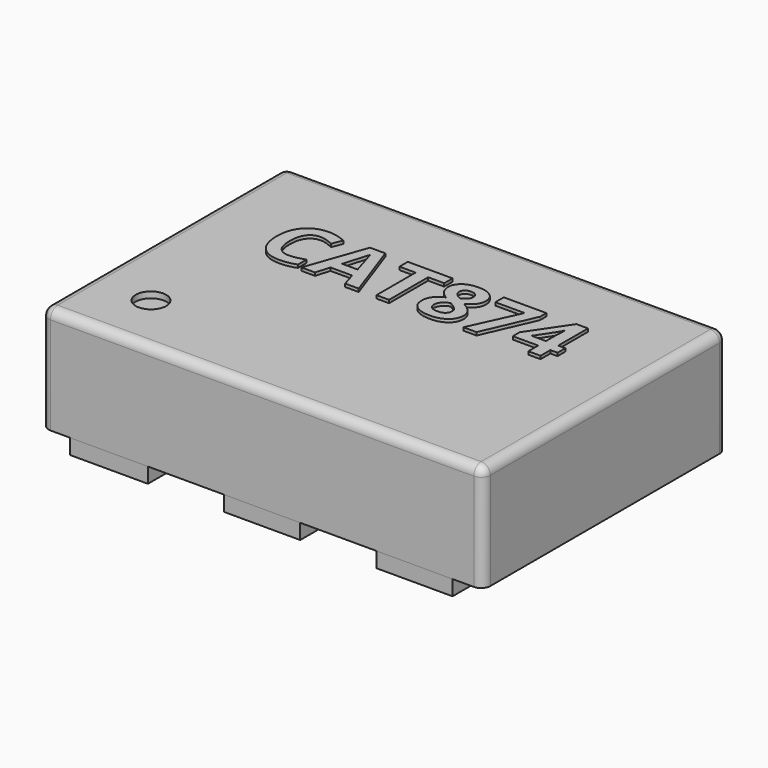
from build123d import *

# Parameters (mm, degrees)
F0_W         = 1.45
F0_H         = 1
F1_DEPTH     = 0.35
F2_R         = 0.05
F3_DEPTH     = 0.02
F4_W         = 0.25
F4_H         = 0.35
F5_DEPTH     = 0.05
F4_W_2       = 0.2562971236
F6_TEXT_SIZE = 0.2726420721
F7_DEPTH     = 0.01
F8_R         = 0.03


# Not quite as in the source:
# - Text() gives the source's letters only with a copy of the font that has no kerning and outlines rounded to 1/6400 em; it was checked with that copy


with BuildPart() as f1:
    # F0 (on Top) → F1 (new body)
    with BuildSketch(Plane.XY):
        Rectangle(F0_W, F0_H)
    extrude(amount=F1_DEPTH)

    # F2 (on face) → F3 (cut)
    with BuildSketch(Plane.XY.offset(0.35)):
        with Locations((-0.525, -0.3)):
            Circle(F2_R)
    extrude(amount=-F3_DEPTH, mode=Mode.SUBTRACT)

    # F8
    f8_edges = [f1.edges().sort_by_distance(p)[0] for p in [
        (0, -0.5, 0.35),
        (0.725, 0, 0.35),
        (0, 0.5, 0.35),
        (-0.725, 0, 0.35),
        (0.725, -0.5, 0.175),
        (0.725, 0.5, 0.175),
        (-0.725, 0.5, 0.175),
        (-0.725, -0.5, 0.175),
    ]]
    fillet(f8_edges, radius=F8_R)


with BuildPart() as f5:
    # F4 (on face) → F5 (new body)
    with BuildSketch(Plane(origin=(0, 0, 0), x_dir=(1, 0, 0), z_dir=(0, 0, -1))):
        with Locations((0, 0.325)):
            Rectangle(F4_W, F4_H)
    extrude(amount=F5_DEPTH)


with BuildPart() as f5b:
    # F4 (on face) → F5, piece 2 (new body)
    with BuildSketch(Plane(origin=(0, 0, 0), x_dir=(1, 0, 0), z_dir=(0, 0, -1))):
        with Locations((0, -0.325)):
            Rectangle(F4_W, F4_H)
    extrude(amount=F5_DEPTH)


with BuildPart() as f5c:
    # F4 (on face) → F5, piece 3 (new body)
    with BuildSketch(Plane(origin=(0, 0, 0), x_dir=(1, 0, 0), z_dir=(0, 0, -1))):
        with Locations((0.5, 0.325)):
            Rectangle(F4_W, F4_H)
    extrude(amount=F5_DEPTH)


with BuildPart() as f5d:
    # F4 (on face) → F5, piece 4 (new body)
    with BuildSketch(Plane(origin=(0, 0, 0), x_dir=(1, 0, 0), z_dir=(0, 0, -1))):
        with Locations((0.5, -0.325)):
            Rectangle(F4_W, F4_H)
    extrude(amount=F5_DEPTH)


with BuildPart() as f5e:
    # F4 (on face) → F5, piece 5 (new body)
    with BuildSketch(Plane(origin=(0, 0, 0), x_dir=(1, 0, 0), z_dir=(0, 0, -1))):
        Polygon((-0.375, 0.15), (-0.375, 0.5), (-0.6312971236, 0.5), (-0.6312971236, 0.2), (-0.5812971236, 0.15), align=None)
        Polygon((-0.375, 0.1), (-0.375, 0.15), (-0.5812971236, 0.15), (-0.5312971236, 0.1), align=None)
    extrude(amount=F5_DEPTH)


with BuildPart() as f5f:
    # F4 (on face) → F5, piece 6 (new body)
    with BuildSketch(Plane(origin=(0, 0, 0), x_dir=(1, 0, 0), z_dir=(0, 0, -1))):
        with Locations((-0.5031485618, -0.325)):
            Rectangle(F4_W_2, F4_H)
    extrude(amount=F5_DEPTH)


with BuildPart() as f7:
    # F6 (on face) → F7 (new body)
    with BuildSketch(Plane.XY.offset(0.35)):
        with Locations((-0.5, 0.068889558)):
            Text('CAT874', F6_TEXT_SIZE, font='Open Sans', font_style=FontStyle.BOLD, text_align=(TextAlign.LEFT, TextAlign.BOTTOM))
    extrude(amount=F7_DEPTH)


solid = Compound([f1.part, f5.part, f5b.part, f5c.part, f5d.part, f5e.part, f5f.part, f7.part])
